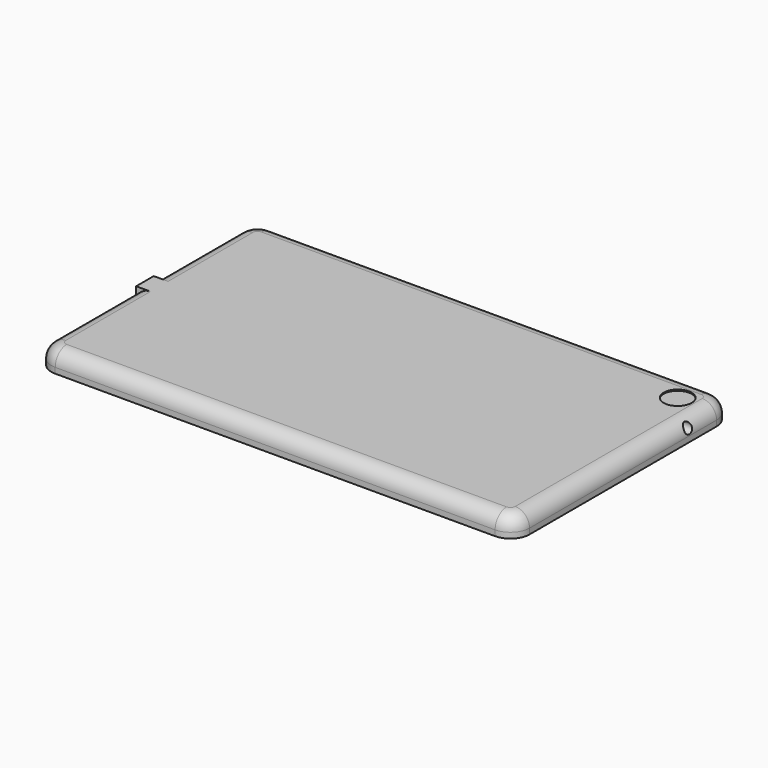
from build123d import *

# Parameters (mm, degrees)
F0_W      = 200
F0_H      = 113.8
F1_DEPTH  = 8.35
F2_R      = 8
F3_R      = 6
F5_R      = 5.85
F6_DEPTH  = 0.5
F8_R      = 2
F9_DEPTH  = 10
F12_W     = 9.2
F12_H     = 5.3
F13_DEPTH = 25


with BuildPart() as f1:
    # F0 (on Top) → F1 (new body)
    with BuildSketch(Plane.XY):
        Rectangle(F0_W, F0_H)
    extrude(amount=F1_DEPTH)

    # F2
    f2_edges = [f1.edges().sort_by_distance(p)[0] for p in [
        (-100, -56.9, 4.175),
        (100, -56.9, 4.175),
        (-100, 56.9, 4.175),
        (100, 56.9, 4.175),
    ]]
    fillet(f2_edges, radius=F2_R)

    # F3
    f3_edges = [f1.edges().sort_by_distance(p)[0] for p in [
        (100, 0, 8.35),
        (97.656854, -54.556854, 8.35),
        (97.656854, 54.556854, 8.35),
        (0, -56.9, 8.35),
        (0, 56.9, 8.35),
        (-97.656854, -54.556854, 8.35),
        (-97.656854, 54.556854, 8.35),
    ]]
    fillet(f3_edges, radius=F3_R)

    # F5 (on face) → F6 (cut)
    with BuildSketch(Plane(origin=(0, 0, 8.35), x_dir=(1, 0, 0), z_dir=(0, 0, -1))):
        with Locations((87.4, -44.3)):
            Circle(F5_R)
    extrude(amount=F6_DEPTH, mode=Mode.SUBTRACT)

    # F8 (on face) → F9 (cut)
    with BuildSketch(Plane(origin=(100, 0, 0), x_dir=(0, -1, 0), z_dir=(-1, 0, 0))):
        with Locations((-34.6, 4.9)):
            Circle(F8_R)
    extrude(amount=F9_DEPTH, mode=Mode.SUBTRACT)

    # F12 (on face) → F13 (join)
    with BuildSketch(Plane.YZ.offset(-100)):
        with Locations((0, 5.7)):
            Rectangle(F12_W, F12_H)
    extrude(amount=F13_DEPTH)


solid = f1.part
